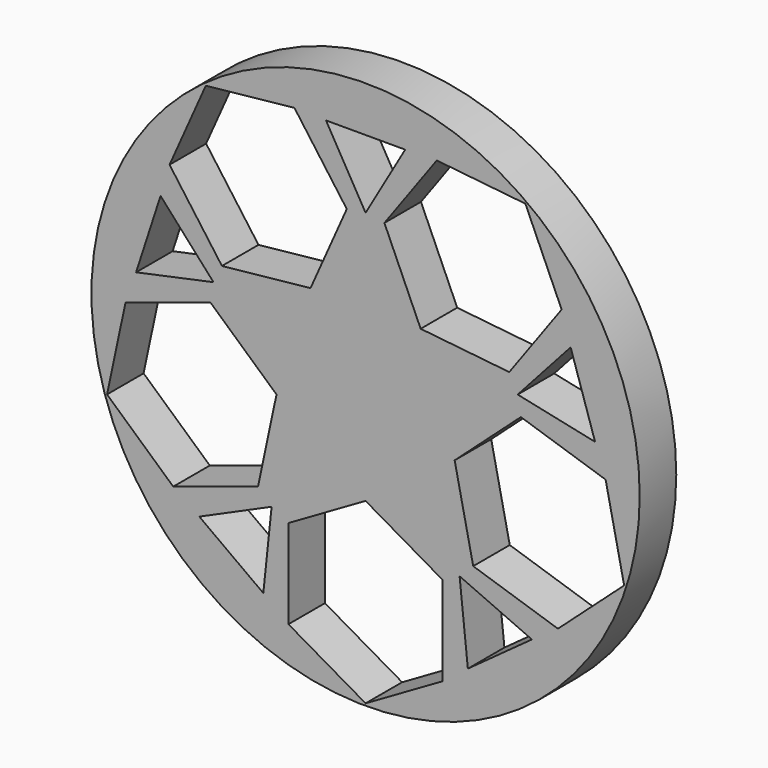
from build123d import *

# Parameters (mm, degrees)
F0_R     = 152.4
F2_DEPTH = 25.4


# Not quite as in the source:
# - a feature of the source that left no trace in its solid (it failed there, or was rolled back) is left out


with BuildPart() as f2:
    # F0 (on Front) → F2 (new body)
    with BuildSketch(Plane.XZ):
        Circle(F0_R)
        Polygon((-52.2541089288, -71.9216107999), (-56.8527436029, -115.6746970812), (-92.4447104794, -89.8156194901), align=None, mode=Mode.SUBTRACT)
        Polygon((-59.8193788497, -64.5381655614), (-106.9252081018, -79.8437772928), (-143.7331713077, -46.7017383599), (-133.4353052615, 1.7459123045), (-86.3294760094, 17.0515240359), (-49.5215128035, -16.0905148971), align=None, mode=Mode.SUBTRACT)
        Polygon((42.8942382494, -76.835), (42.8942382494, -126.365), (0, -151.13), (-42.8942382494, -126.365), (-42.8942382494, -76.835), (0, -52.07), align=None, mode=Mode.SUBTRACT)
        Polygon((52.2541089288, -71.9216107999), (92.4447104794, -89.8156194901), (56.8527436029, -115.6746970812), align=None, mode=Mode.SUBTRACT)
        Polygon((86.3294760094, 17.0515240359), (133.4353052615, 1.7459123045), (143.7331713077, -46.7017383599), (106.9252081018, -79.8437772928), (59.8193788497, -64.5381655614), (49.5215128035, -16.0905148971), align=None, mode=Mode.SUBTRACT)
        Polygon((-84.5489242986, 27.4716107999), (-127.5816383797, 18.3247250555), (-113.9867167593, 60.1655915157), align=None, mode=Mode.SUBTRACT)
        Polygon((-79.8646475645, 36.9482201115), (-108.9776511105, 77.0188318428), (-88.831985179, 122.2667383599), (-39.5733157014, 127.4440331455), (-10.4603121553, 87.3734214141), (-30.6059780869, 42.1255148971), align=None, mode=Mode.SUBTRACT)
        Polygon((84.5489242986, 27.4716107999), (113.9867167593, 60.1655915157), (127.5816383797, 18.3247250555), align=None, mode=Mode.SUBTRACT)
        Polygon((21.9970452561, 127), (0, 88.9), (-21.9970452561, 127), align=None, mode=Mode.SUBTRACT)
        Polygon((10.4603121553, 87.3734214141), (39.5733157014, 127.4440331455), (88.831985179, 122.2667383599), (108.9776511105, 77.0188318428), (79.8646475645, 36.9482201115), (30.6059780869, 42.1255148971), align=None, mode=Mode.SUBTRACT)
    extrude(amount=F2_DEPTH)


solid = f2.part
